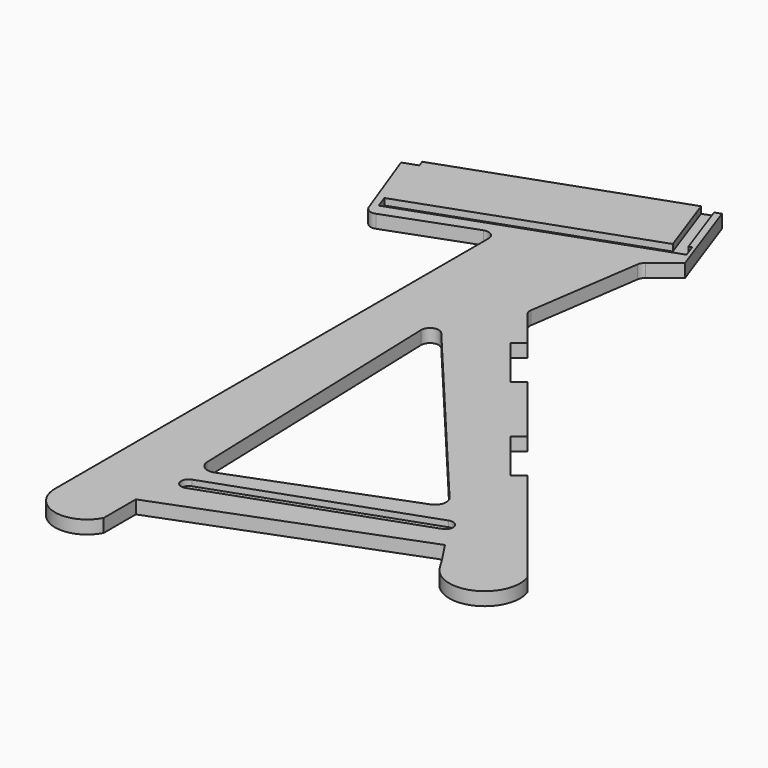
from build123d import *

# Parameters (mm, degrees)
F1_DEPTH = 19.05
F3_DEPTH = 8.4666582
F5_DEPTH = 9.525
F6_W     = 94.742
F6_H     = 19.05
F7_DEPTH = 19.05


# Not quite as in the source:
# - a feature names something its author has since deleted; it is built from what else it names


with BuildPart() as f1:
    # F0 (on Top) → F1 (new body)
    with BuildSketch(Plane.XY):
        with BuildLine():
            Line((732.4377516272, 429.8118038565), (732.4377516272, -265.5463867273))
            ThreePointArc((732.4377516272, -265.5463867273), (767.5922703415, -310.3140075425), (819.4192408881, -286.7779674454))
            Line((819.4192408881, -286.7779674454), (819.4192408881, -229.1199674454))
            Line((819.4192408881, -229.1199674454), (1159.4623036636, -98.9686407408))
            Line((1159.4623036636, -98.9686407408), (1178.6487772739, -128.0367093729))
            Line((1178.6487772739, -128.0367093729), (1189.3036458742, -145.3996676047))
            ThreePointArc((1189.3036458742, -145.3996676047), (1254.3589120262, -165.180351508), (1280.8355912672, -102.5508970465))
            Line((1280.8355912672, -102.5508970465), (881.2480453078, 396.8848219998))
            ThreePointArc((881.2480453078, 396.8848219998), (878.9075846932, 401.4943033077), (878.5980767553, 406.6546597539))
            Line((878.5980767553, 406.6546597539), (902.2401524871, 568.497452094))
            ThreePointArc((902.2401524871, 568.497452094), (903.8120375637, 573.0182606597), (906.9455405898, 576.6362285378))
            Line((906.9455405898, 576.6362285378), (941.9003890149, 604.1852707886))
            Line((941.9003890149, 604.1852707886), (899.3018677789, 723.8279303566))
            Line((899.3018677789, 723.8279303566), (891.7270738587, 721.1309406639))
            Line((891.7270738587, 721.1309406639), (888.532184766, 730.1041401315))
            Line((888.532184766, 730.1041401315), (557.8398737201, 612.361827435))
            Line((557.8398737201, 612.361827435), (561.0347628128, 603.3886279674))
            Line((561.0347628128, 603.3886279674), (540.3738890749, 596.0323666485))
            Line((540.3738890749, 596.0323666485), (579.8650741531, 488.7713005475))
            ThreePointArc((579.8650741531, 488.7713005475), (586.4584656719, 481.6292642269), (596.1708798397, 481.2413137672))
            Line((596.1708798397, 481.2413137672), (715.3498421741, 525.1204082985))
            ThreePointArc((715.3498421741, 525.1204082985), (727.0028583004, 523.6192401995), (732.4377516272, 513.202512065))
            Line((732.4377516272, 513.202512065), (732.4377516272, 429.8118038565))
        make_face()
        with BuildLine():
            ThreePointArc((847.6172180507, -123.0333171416), (832.579476833, -121.3659760987), (825.2142352601, -108.1498153983))
            Line((825.2142352601, -108.1498153983), (812.2279623998, 291.9047427935))
            ThreePointArc((812.2279623998, 291.9047427935), (820.3847868922, 304.1789193457), (834.6503380579, 300.4798321914))
            Line((834.6503380579, 300.4798321914), (1091.877202569, -6.0938706764))
            ThreePointArc((1091.877202569, -6.0938706764), (1095.2114543488, -20.8476640537), (1085.1310970041, -32.1249886369))
            Line((1085.1310970041, -32.1249886369), (847.6172180507, -123.0333171416))
        make_face(mode=Mode.SUBTRACT)
    extrude(amount=F1_DEPTH)

    # F2 (on face) → F3 (cut)
    with BuildSketch(Plane.XY.offset(19.05)):
        with BuildLine():
            ThreePointArc((838.451528287, -152.2525984903), (831.9027765287, -166.0430988586), (845.6932768971, -172.5918506169))
            Line((845.6932768971, -172.5918506169), (1132.8356598603, -70.3553996504))
            ThreePointArc((1132.8356598603, -70.3553996504), (1139.3844116185, -56.564899282), (1125.5939112501, -50.0161475238))
            Line((1125.5939112501, -50.0161475238), (838.451528287, -152.2525984903))
        make_face()
    extrude(amount=-F3_DEPTH, mode=Mode.SUBTRACT)

    # F4 (on face) → F5 (cut)
    with BuildSketch(Plane.XY.offset(19.05)):
        Polygon((579.7007303012, 517.0436017545), (586.2609025716, 498.618632181), (926.4367371726, 619.7375338049), (930.6009060633, 621.2201775171), (924.161381266, 639.3062953154), (919.9972123753, 637.8236516032), (891.8491444715, 716.8806143331), (890.4923506062, 720.6913200061), (891.7270738587, 721.1309406639), (888.532184766, 730.1041401315), (869.645537074, 723.3795883228), (874.197220032, 710.5956831823), (902.2246404628, 631.8775722275), align=None)
    extrude(amount=-F5_DEPTH, mode=Mode.SUBTRACT)

    # F6 (on face) → F7 (cut)
    with BuildSketch(Plane(origin=(730.9119602838, 584.7866009261, 0), x_dir=(-0.6247321984, 0.7808390873, 0), z_dir=(0.7808390873, 0.6247321984, 0))):
        with Locations((-357.880134458, 9.525)):
            Rectangle(F6_W, F6_H)
        with Locations((-584.981534458, 9.525)):
            Rectangle(F6_W, F6_H)
    extrude(amount=-F7_DEPTH, mode=Mode.SUBTRACT)


solid = f1.part
